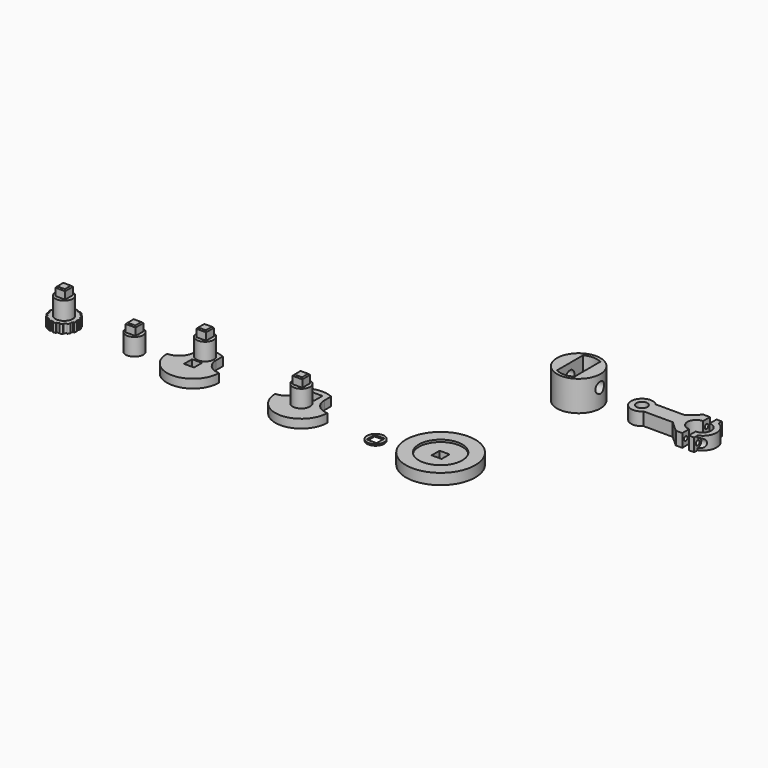
from build123d import *

# Parameters (mm, degrees)
F0_R       = 2.5
F1_DEPTH   = 6
F3_D       = 2.2
F4_R       = 2.1
F5_DEPTH   = 25
F0_R_2     = 10
F6_DEPTH   = 3
F7_R       = 10
F8_DEPTH   = 11
F10_D      = 2
F10_DEPTH  = 3
F10_TIP    = 0.600860619
F0_R_3     = 4
F0_W       = 4.5
F0_H       = 4.5
F11_DEPTH  = 12
F0_W_2     = 4.6
F0_H_2     = 4.6
F12_DEPTH  = 4
F13_DEPTH  = 15.9
F14_DEPTH  = 12
F15_DEPTH  = 4
F16_DEPTH  = 11.9
F17_DEPTH  = 8
F18_DEPTH  = 15.9
F0_R_4     = 16
F19_DEPTH  = 4
F20_R      = 16
F20_R_2    = 10
F21_DEPTH  = 1
F22_DEPTH  = 0.7
F23_DEPTH  = 16.1
F24_DEPTH  = 12.2
F25_DEPTH  = 4
F26_SIZE   = 0.5
F26_2_SIZE = 0.5
F26_3_SIZE = 0.5
F26_4_SIZE = 0.5
F28_D      = 5
F28_DEPTH  = 15
F28_TIP    = 1.5021515476
F29_D      = 5
F29_DEPTH  = 10
F29_TIP    = 1.5021515476


with BuildPart() as f1:
    # F0 (on Top) → F1 (new body)
    with BuildSketch(Plane.XY):
        with BuildLine():
            Line((39.7844910622, 54.6768961251), (39.7844910622, 58.6768961251))
            ThreePointArc((39.7844910622, 58.6768961251), (35.7844910622, 62.6768961251), (39.7844910622, 66.6768961251))
            Line((39.7844910622, 66.6768961251), (39.7844910622, 70.6768961251))
            Line((39.7844910622, 70.6768961251), (36.7844910622, 70.6768961251))
            Line((36.7844910622, 70.6768961251), (31.7844910622, 66.1768961251))
            Line((31.7844910622, 66.1768961251), (18.3552052764, 66.1768961251))
            ThreePointArc((18.3552052764, 66.1768961251), (9.7844910622, 62.6768961251), (18.3552052764, 59.1768961251))
            Line((18.3552052764, 59.1768961251), (31.7844910622, 59.1768961251))
            Line((31.7844910622, 59.1768961251), (36.7844910622, 54.6768961251))
            Line((36.7844910622, 54.6768961251), (39.7844910622, 54.6768961251))
        make_face()
        with Locations((14.7844910622, 62.6768961251)):
            Circle(F0_R, mode=Mode.SUBTRACT)
    extrude(amount=F1_DEPTH)

    # F10
    with Locations(Plane.YZ.offset(39.7844910622)):
        with Locations((56.6768961251, 3), (68.6768961251, 3)):
            Hole(F10_D / 2, depth=F10_DEPTH)
            with Locations((0, 0, -(F10_DEPTH + F10_TIP / 2))):  # 118° drill point
                Cone(0, F10_D / 2, F10_TIP, mode=Mode.SUBTRACT)


with BuildPart() as f1b:
    # F0 (on Top) → F1, piece 2 (new body)
    with BuildSketch(Plane.XY):
        with BuildLine():
            Line((42.7844910622, 69.1768961251), (42.7844910622, 66.6768961251))
            ThreePointArc((42.7844910622, 66.6768961251), (46.7844910622, 62.6768961251), (42.7844910622, 58.6768961251))
            Line((42.7844910622, 58.6768961251), (42.7844910622, 56.1768961251))
            ThreePointArc((42.7844910622, 56.1768961251), (44.0592459406, 56.3031217331), (45.2844910622, 56.6768961251))
            ThreePointArc((45.2844910622, 56.6768961251), (49.2844910622, 62.6768961251), (45.2844910622, 68.6768961251))
            ThreePointArc((45.2844910622, 68.6768961251), (44.0592459406, 69.0506705171), (42.7844910622, 69.1768961251))
        make_face()
        with BuildLine():
            Line((42.7844910622, 70.6768961251), (42.7844910622, 69.1768961251))
            ThreePointArc((42.7844910622, 69.1768961251), (44.0592459406, 69.0506705171), (45.2844910622, 68.6768961251))
            Line((45.2844910622, 68.6768961251), (45.2844910622, 70.6768961251))
            Line((45.2844910622, 70.6768961251), (42.7844910622, 70.6768961251))
        make_face()
        with BuildLine():
            ThreePointArc((45.2844910622, 56.6768961251), (44.0592459406, 56.3031217331), (42.7844910622, 56.1768961251))
            Line((42.7844910622, 56.1768961251), (42.7844910622, 54.6768961251))
            Line((42.7844910622, 54.6768961251), (45.2844910622, 54.6768961251))
            Line((45.2844910622, 54.6768961251), (45.2844910622, 56.6768961251))
        make_face()
    extrude(amount=F1_DEPTH)

    # F3 (through all)
    with Locations(Plane(origin=(42.7844910622, 0, 0), x_dir=(0, -1, 0), z_dir=(-1, 0, 0))):
        with Locations((-68.6768961251, 3), (-56.6768961251, 3)):
            Hole(F3_D / 2)

    # F4 (on face) → F5 (cut)
    with BuildSketch(Plane.YZ.offset(45.2844910622)):
        with Locations((56.6768961251, 2.963399974)):
            Circle(F4_R)
        with BuildLine():
            Line((68.6768961251, 4.1), (68.6768961251, 5.063143551))
            ThreePointArc((68.6768961251, 5.063143551), (66.6097124413, 2.963399974), (68.6768961251, 0.8636563969))
            Line((68.6768961251, 0.8636563969), (68.6768961251, 1.9))
            ThreePointArc((68.6768961251, 1.9), (69.7768961251, 3), (68.6768961251, 4.1))
        make_face()
    extrude(amount=F5_DEPTH, mode=Mode.SUBTRACT)


with BuildPart() as f6:
    # F0 (on Top) → F6 (new body)
    with BuildSketch(Plane.XY):
        with Locations((-12.4482074752, 60.2258183062)):
            Circle(F0_R_2)
    extrude(amount=F6_DEPTH)

    # F7 (on face) → F8 (join)
    with BuildSketch(Plane.XY.offset(3)):
        with Locations((-12.4482074752, 60.2258183062)):
            Circle(F7_R)
        with BuildLine():
            ThreePointArc((-8.4482074752, 67.7258183062), (-5.1595176067, 64.5990322273), (-3.9482074752, 60.2258183062))
            ThreePointArc((-3.9482074752, 60.2258183062), (-5.1595176067, 55.8526043851), (-8.4482074752, 52.7258183062))
            ThreePointArc((-8.4482074752, 52.7258183062), (-12.4482074752, 51.7258183062), (-16.4482074752, 52.7258183062))
            ThreePointArc((-16.4482074752, 52.7258183062), (-20.9482074752, 60.2258183062), (-16.4482074752, 67.7258183062))
            ThreePointArc((-16.4482074752, 67.7258183062), (-12.4482074752, 68.7258183062), (-8.4482074752, 67.7258183062))
        make_face(mode=Mode.SUBTRACT)
        with BuildLine():
            Line((-16.4482074752, 52.7258183062), (-16.4482074752, 67.7258183062))
            ThreePointArc((-16.4482074752, 67.7258183062), (-20.9482074752, 60.2258183062), (-16.4482074752, 52.7258183062))
        make_face()
        with BuildLine():
            ThreePointArc((-8.4482074752, 52.7258183062), (-5.1595176067, 55.8526043851), (-3.9482074752, 60.2258183062))
            ThreePointArc((-3.9482074752, 60.2258183062), (-5.1595176067, 64.5990322273), (-8.4482074752, 67.7258183062))
            Line((-8.4482074752, 67.7258183062), (-8.4482074752, 52.7258183062))
        make_face()
    extrude(amount=F8_DEPTH)

    # F28 (one way)
    with BuildSketch(Plane(origin=(-8.4482074752, 0, 0), x_dir=(0, -1, 0), z_dir=(1, 0, 0))):
        with Locations((-60.2258183062, -8.5)):
            Circle(F28_D / 2)
    extrude(amount=-F28_DEPTH, mode=Mode.SUBTRACT)
    with Locations(Plane(origin=(-8.4482074752, 0, 0), x_dir=(0, -1, 0), z_dir=(1, 0, 0))):
        with Locations((-60.2258183062, -8.5)):
            with Locations((0, 0, -(F28_DEPTH + F28_TIP / 2))):  # 118° drill point
                Cone(0, F28_D / 2, F28_TIP, mode=Mode.SUBTRACT)

    # F29
    with Locations(Plane(origin=(-8.4482074752, 0, 0), x_dir=(0, -1, 0), z_dir=(-1, 0, 0))):
        with Locations((-60.2258183062, 8.5)):
            Hole(F29_D / 2, depth=F29_DEPTH)
            with Locations((0, 0, -(F29_DEPTH + F29_TIP / 2))):  # 118° drill point
                Cone(0, F29_D / 2, F29_TIP, mode=Mode.SUBTRACT)


with BuildPart() as f11:
    # F0 (on Top) → F11 (new body)
    with BuildSketch(Plane.XY):
        with Locations((-134.2660826899, -3)):
            Circle(F0_R_3)
        with Locations((-134.2660826899, -3)):
            Rectangle(F0_W, F0_H, mode=Mode.SUBTRACT)
    extrude(amount=F11_DEPTH)

    # F0 (on Top) → F12 (join)
    with BuildSketch(Plane.XY):
        with BuildLine():
            ThreePointArc((-146.2660826899, -10), (-134.2660826899, -22), (-122.2660826899, -10))
            ThreePointArc((-122.2660826899, -10), (-127.2158301582, -7.9497474683), (-129.2660826899, -3))
            Line((-129.2660826899, -3), (-129.2660826899, 0.9087121146))
            ThreePointArc((-129.2660826899, 0.9087121146), (-134.2660826899, 2), (-139.2660826899, 0.9087121146))
            Line((-139.2660826899, 0.9087121146), (-139.2660826899, -3))
            ThreePointArc((-139.2660826899, -3), (-141.3163352216, -7.9497474683), (-146.2660826899, -10))
        make_face()
        with Locations((-134.2660826899, -10)):
            Rectangle(F0_W_2, F0_H_2, mode=Mode.SUBTRACT)
        with Locations((-134.2660826899, -3)):
            Circle(F0_R_3, mode=Mode.SUBTRACT)
    extrude(amount=F12_DEPTH)

    # F0 (on Top) → F13 (join)
    with BuildSketch(Plane.XY):
        with Locations((-134.2660826899, -3)):
            Rectangle(F0_W, F0_H)
    extrude(amount=F13_DEPTH)

    # F26
    f26_edges = [f11.edges().sort_by_distance(p)[0] for p in [
        (-132.016083, -3, 15.9),
        (-134.266083, -0.75, 15.9),
        (-136.516083, -3, 15.9),
        (-134.266083, -5.25, 15.9),
    ]]
    chamfer(f26_edges, length=F26_SIZE)


with BuildPart() as f14:
    # F0 (on Top) → F14 (new body)
    with BuildSketch(Plane.XY):
        with Locations((-84.2660826899, -10)):
            Circle(F0_R_3)
        with Locations((-84.2660826899, -10)):
            Rectangle(F0_W, F0_H, mode=Mode.SUBTRACT)
    extrude(amount=F14_DEPTH)

    # F0 (on Top) → F15 (join)
    with BuildSketch(Plane.XY):
        with BuildLine():
            ThreePointArc((-96.2660826899, -10), (-84.2660826899, -22), (-72.2660826899, -10))
            ThreePointArc((-72.2660826899, -10), (-77.2158301582, -7.9497474683), (-79.2660826899, -3))
            Line((-79.2660826899, -3), (-79.2660826899, 0.9087121146))
            ThreePointArc((-79.2660826899, 0.9087121146), (-84.2660826899, 2), (-89.2660826899, 0.9087121146))
            Line((-89.2660826899, 0.9087121146), (-89.2660826899, -3))
            ThreePointArc((-89.2660826899, -3), (-91.3163352216, -7.9497474683), (-96.2660826899, -10))
        make_face()
        with Locations((-84.2660826899, -10)):
            Circle(F0_R_3, mode=Mode.SUBTRACT)
        with Locations((-84.2660826899, -3)):
            Rectangle(F0_W_2, F0_H_2, mode=Mode.SUBTRACT)
    extrude(amount=F15_DEPTH)

    # F0 (on Top) → F18 (join)
    with BuildSketch(Plane.XY):
        with Locations((-84.2660826899, -10)):
            Rectangle(F0_W, F0_H)
    extrude(amount=F18_DEPTH)

    # F26#2
    f26_2_edges = [f14.edges().sort_by_distance(p)[0] for p in [
        (-82.016083, -10, 15.9),
        (-84.266083, -7.75, 15.9),
        (-86.516083, -10, 15.9),
        (-84.266083, -12.25, 15.9),
    ]]
    chamfer(f26_2_edges, length=F26_2_SIZE)


with BuildPart() as f16:
    # F0 (on Top) → F16 (new body)
    with BuildSketch(Plane.XY):
        with Locations((-161.2660826899, -10)):
            Rectangle(F0_W, F0_H)
    extrude(amount=F16_DEPTH)

    # F0 (on Top) → F17 (join)
    with BuildSketch(Plane.XY):
        with Locations((-161.2660826899, -10)):
            Circle(F0_R_3)
        with Locations((-161.2660826899, -10)):
            Rectangle(F0_W, F0_H, mode=Mode.SUBTRACT)
    extrude(amount=F17_DEPTH)

    # F26#3
    f26_3_edges = [f16.edges().sort_by_distance(p)[0] for p in [
        (-161.266083, -12.25, 11.9),
        (-159.016083, -10, 11.9),
        (-161.266083, -7.75, 11.9),
        (-163.516083, -10, 11.9),
    ]]
    chamfer(f26_3_edges, length=F26_3_SIZE)


with BuildPart() as f19:
    # F0 (on Top) → F19 (new body)
    with BuildSketch(Plane.XY):
        with Locations((-20, -10)):
            Circle(F0_R_4)
        with Locations((-20, -10)):
            Rectangle(F0_W_2, F0_H_2, mode=Mode.SUBTRACT)
    extrude(amount=F19_DEPTH)

    # F20 (on face) → F21 (join)
    with BuildSketch(Plane.XY.offset(4)):
        with Locations((-20, -10)):
            Circle(F20_R)
        with Locations((-20, -10)):
            Circle(F20_R_2, mode=Mode.SUBTRACT)
    extrude(amount=F21_DEPTH)


with BuildPart() as f22:
    # F0 (on Top) → F22 (new body)
    with BuildSketch(Plane.XY):
        with Locations((-50, -10)):
            Circle(F0_R_3)
        with Locations((-50, -10)):
            Rectangle(F0_W_2, F0_H_2, mode=Mode.SUBTRACT)
    extrude(amount=F22_DEPTH)


with BuildPart() as f23:
    # F0 (on Top) → F23 (new body)
    with BuildSketch(Plane.XY):
        with Locations((-193.7630802393, -10)):
            Rectangle(F0_W, F0_H)
    extrude(amount=F23_DEPTH)

    # F0 (on Top) → F24 (join)
    with BuildSketch(Plane.XY):
        with Locations((-193.7630802393, -10)):
            Circle(F0_R_3)
        with Locations((-193.7630802393, -10)):
            Rectangle(F0_W, F0_H, mode=Mode.SUBTRACT)
    extrude(amount=F24_DEPTH)

    # F0 (on Top) → F25 (join)
    with BuildSketch(Plane.XY):
        with BuildLine():
            ThreePointArc((-187.7959488671, -10.6271707796), (-187.7713030308, -10.3140157375), (-187.7630802393, -10))
            ThreePointArc((-187.7630802393, -10), (-187.7713030308, -9.6859842625), (-187.7959488671, -9.3728292204))
            ThreePointArc((-187.7959488671, -9.3728292204), (-187.8941946349, -8.7525298551), (-188.0567411415, -8.1458980338))
            ThreePointArc((-188.0567411415, -8.1458980338), (-188.2818074934, -7.5595801415), (-188.5669278166, -7))
            ThreePointArc((-188.5669278166, -7), (-188.908978273, -6.4732884862), (-189.3042112864, -5.9852163618))
            ThreePointArc((-189.3042112864, -5.9852163618), (-189.7482966011, -5.5411310471), (-190.2363687255, -5.1458980338))
            ThreePointArc((-190.2363687255, -5.1458980338), (-190.7630802393, -4.8038475773), (-191.3226603808, -4.5187272541))
            ThreePointArc((-191.3226603808, -4.5187272541), (-191.908978273, -4.2936609022), (-192.5156100944, -4.1311143956))
            ThreePointArc((-192.5156100944, -4.1311143956), (-193.1359094597, -4.0328686278), (-193.7630802393, -4))
            ThreePointArc((-193.7630802393, -4), (-194.3902510189, -4.0328686278), (-195.0105503842, -4.1311143956))
            ThreePointArc((-195.0105503842, -4.1311143956), (-195.6171822055, -4.2936609022), (-196.2035000978, -4.5187272541))
            ThreePointArc((-196.2035000978, -4.5187272541), (-196.7630802393, -4.8038475773), (-197.2897917531, -5.1458980338))
            ThreePointArc((-197.2897917531, -5.1458980338), (-197.7778638774, -5.5411310471), (-198.2219491922, -5.9852163618))
            ThreePointArc((-198.2219491922, -5.9852163618), (-198.6171822055, -6.4732884862), (-198.959232662, -7))
            ThreePointArc((-198.959232662, -7), (-199.2443529852, -7.5595801415), (-199.4694193371, -8.1458980338))
            ThreePointArc((-199.4694193371, -8.1458980338), (-199.6319658437, -8.7525298551), (-199.7302116115, -9.3728292204))
            ThreePointArc((-199.7302116115, -9.3728292204), (-199.7630802393, -10), (-199.7302116115, -10.6271707796))
            ThreePointArc((-199.7302116115, -10.6271707796), (-199.6319658437, -11.2474701449), (-199.4694193371, -11.8541019662))
            ThreePointArc((-199.4694193371, -11.8541019662), (-199.2443529852, -12.4404198585), (-198.959232662, -13))
            ThreePointArc((-198.959232662, -13), (-198.6171822055, -13.5267115138), (-198.2219491922, -14.0147836382))
            ThreePointArc((-198.2219491922, -14.0147836382), (-197.7778638774, -14.4588689529), (-197.2897917531, -14.8541019662))
            ThreePointArc((-197.2897917531, -14.8541019662), (-196.7630802393, -15.1961524227), (-196.2035000978, -15.4812727459))
            ThreePointArc((-196.2035000978, -15.4812727459), (-195.6171822055, -15.7063390978), (-195.0105503842, -15.8688856044))
            ThreePointArc((-195.0105503842, -15.8688856044), (-194.3902510189, -15.9671313722), (-193.7630802393, -16))
            ThreePointArc((-193.7630802393, -16), (-193.1359094597, -15.9671313722), (-192.5156100944, -15.8688856044))
            ThreePointArc((-192.5156100944, -15.8688856044), (-191.908978273, -15.7063390978), (-191.3226603808, -15.4812727459))
            ThreePointArc((-191.3226603808, -15.4812727459), (-190.7630802393, -15.1961524227), (-190.2363687255, -14.8541019662))
            ThreePointArc((-190.2363687255, -14.8541019662), (-189.7482966011, -14.4588689529), (-189.3042112864, -14.0147836382))
            ThreePointArc((-189.3042112864, -14.0147836382), (-188.908978273, -13.5267115138), (-188.5669278166, -13))
            ThreePointArc((-188.5669278166, -13), (-188.2818074934, -12.4404198585), (-188.0567411415, -11.8541019662))
            ThreePointArc((-188.0567411415, -11.8541019662), (-187.8941946349, -11.2474701449), (-187.7959488671, -10.6271707796))
        make_face()
        with Locations((-193.7630802393, -10)):
            Circle(F0_R_3, mode=Mode.SUBTRACT)
        with BuildLine():
            ThreePointArc((-193.7630802393, -4), (-193.1359094597, -4.0328686278), (-192.5156100944, -4.1311143956))
            Line((-192.5156100944, -4.1311143956), (-192.411654249, -3.6420405952))
            ThreePointArc((-192.411654249, -3.6420405952), (-193.0836452281, -3.5356076801), (-193.7630802393, -3.5))
            Line((-193.7630802393, -3.5), (-193.7630802393, -4))
        make_face()
        with BuildLine():
            ThreePointArc((-191.3226603808, -4.5187272541), (-190.7630802393, -4.8038475773), (-190.2363687255, -5.1458980338))
            Line((-190.2363687255, -5.1458980338), (-189.9424760994, -4.7413895366))
            ThreePointArc((-189.9424760994, -4.7413895366), (-190.5130802393, -4.3708348754), (-191.1192920593, -4.0619545253))
            Line((-191.1192920593, -4.0619545253), (-191.3226603808, -4.5187272541))
        make_face()
        with BuildLine():
            ThreePointArc((-189.3042112864, -5.9852163618), (-188.908978273, -6.4732884862), (-188.5669278166, -7))
            Line((-188.5669278166, -7), (-188.1339151147, -6.75))
            ThreePointArc((-188.1339151147, -6.75), (-188.5044697759, -6.1793958601), (-188.9326388737, -5.6506510587))
            Line((-188.9326388737, -5.6506510587), (-189.3042112864, -5.9852163618))
        make_face()
        with BuildLine():
            ThreePointArc((-188.0567411415, -8.1458980338), (-187.8941946349, -8.7525298551), (-187.7959488671, -9.3728292204))
            Line((-187.7959488671, -9.3728292204), (-187.2986879194, -9.3205649888))
            ThreePointArc((-187.2986879194, -9.3205649888), (-187.4051208345, -8.6485740097), (-187.5812128834, -7.9913895366))
            Line((-187.5812128834, -7.9913895366), (-188.0567411415, -8.1458980338))
        make_face()
        with BuildLine():
            Line((-187.2986879194, -10.6794350112), (-187.7959488671, -10.6271707796))
            ThreePointArc((-187.7959488671, -10.6271707796), (-187.8941946349, -11.2474701449), (-188.0567411415, -11.8541019662))
            Line((-188.0567411415, -11.8541019662), (-187.5812128834, -12.0086104634))
            ThreePointArc((-187.5812128834, -12.0086104634), (-187.4051208345, -11.3514259903), (-187.2986879194, -10.6794350112))
        make_face()
        with BuildLine():
            Line((-188.1339151147, -13.25), (-188.5669278166, -13))
            ThreePointArc((-188.5669278166, -13), (-188.908978273, -13.5267115138), (-189.3042112864, -14.0147836382))
            Line((-189.3042112864, -14.0147836382), (-188.9326388737, -14.3493489413))
            ThreePointArc((-188.9326388737, -14.3493489413), (-188.5044697759, -13.8206041399), (-188.1339151147, -13.25))
        make_face()
        with BuildLine():
            Line((-189.9424760994, -15.2586104634), (-190.2363687255, -14.8541019662))
            ThreePointArc((-190.2363687255, -14.8541019662), (-190.7630802393, -15.1961524227), (-191.3226603808, -15.4812727459))
            Line((-191.3226603808, -15.4812727459), (-191.1192920593, -15.9380454747))
            ThreePointArc((-191.1192920593, -15.9380454747), (-190.5130802393, -15.6291651246), (-189.9424760994, -15.2586104634))
        make_face()
        with BuildLine():
            Line((-192.411654249, -16.3579594048), (-192.5156100944, -15.8688856044))
            ThreePointArc((-192.5156100944, -15.8688856044), (-193.1359094597, -15.9671313722), (-193.7630802393, -16))
            Line((-193.7630802393, -16), (-193.7630802393, -16.5))
            ThreePointArc((-193.7630802393, -16.5), (-193.0836452281, -16.4643923199), (-192.411654249, -16.3579594048))
        make_face()
        with BuildLine():
            Line((-195.1145062296, -16.3579594048), (-195.0105503842, -15.8688856044))
            ThreePointArc((-195.0105503842, -15.8688856044), (-195.6171822055, -15.7063390978), (-196.2035000978, -15.4812727459))
            Line((-196.2035000978, -15.4812727459), (-196.4068684193, -15.9380454747))
            ThreePointArc((-196.4068684193, -15.9380454747), (-195.7716907027, -16.1818673559), (-195.1145062296, -16.3579594048))
        make_face()
        with BuildLine():
            Line((-197.5836843792, -15.2586104634), (-197.2897917531, -14.8541019662))
            ThreePointArc((-197.2897917531, -14.8541019662), (-197.7778638774, -14.4588689529), (-198.2219491922, -14.0147836382))
            Line((-198.2219491922, -14.0147836382), (-198.5935216049, -14.3493489413))
            ThreePointArc((-198.5935216049, -14.3493489413), (-198.1124291806, -14.8304413656), (-197.5836843792, -15.2586104634))
        make_face()
        with BuildLine():
            Line((-199.3922453639, -13.25), (-198.959232662, -13))
            ThreePointArc((-198.959232662, -13), (-199.2443529852, -12.4404198585), (-199.4694193371, -11.8541019662))
            Line((-199.4694193371, -11.8541019662), (-199.9449475952, -12.0086104634))
            ThreePointArc((-199.9449475952, -12.0086104634), (-199.701125714, -12.64378818), (-199.3922453639, -13.25))
        make_face()
        with BuildLine():
            ThreePointArc((-199.7302116115, -10.6271707796), (-199.7630802393, -10), (-199.7302116115, -9.3728292204))
            Line((-199.7302116115, -9.3728292204), (-200.2274725592, -9.3205649888))
            ThreePointArc((-200.2274725592, -9.3205649888), (-200.2630802393, -10), (-200.2274725592, -10.6794350112))
            Line((-200.2274725592, -10.6794350112), (-199.7302116115, -10.6271707796))
        make_face()
        with BuildLine():
            ThreePointArc((-199.4694193371, -8.1458980338), (-199.2443529852, -7.5595801415), (-198.959232662, -7))
            Line((-198.959232662, -7), (-199.3922453639, -6.75))
            ThreePointArc((-199.3922453639, -6.75), (-199.701125714, -7.35621182), (-199.9449475952, -7.9913895366))
            Line((-199.9449475952, -7.9913895366), (-199.4694193371, -8.1458980338))
        make_face()
        with BuildLine():
            ThreePointArc((-198.2219491922, -5.9852163618), (-197.7778638774, -5.5411310471), (-197.2897917531, -5.1458980338))
            Line((-197.2897917531, -5.1458980338), (-197.5836843792, -4.7413895366))
            ThreePointArc((-197.5836843792, -4.7413895366), (-198.1124291806, -5.1695586344), (-198.5935216049, -5.6506510587))
            Line((-198.5935216049, -5.6506510587), (-198.2219491922, -5.9852163618))
        make_face()
        with BuildLine():
            ThreePointArc((-196.2035000978, -4.5187272541), (-195.6171822055, -4.2936609022), (-195.0105503842, -4.1311143956))
            Line((-195.0105503842, -4.1311143956), (-195.1145062296, -3.6420405952))
            ThreePointArc((-195.1145062296, -3.6420405952), (-195.7716907027, -3.8181326441), (-196.4068684193, -4.0619545253))
            Line((-196.4068684193, -4.0619545253), (-196.2035000978, -4.5187272541))
        make_face()
    extrude(amount=F25_DEPTH)

    # F26#4
    f26_4_edges = [f23.edges().sort_by_distance(p)[0] for p in [
        (-196.01308, -10, 16.1),
        (-193.76308, -7.75, 16.1),
        (-191.51308, -10, 16.1),
        (-193.76308, -12.25, 16.1),
    ]]
    chamfer(f26_4_edges, length=F26_4_SIZE)


solid = Compound([f1.part, f1b.part, f6.part, f11.part, f14.part, f16.part, f19.part, f22.part, f23.part])
